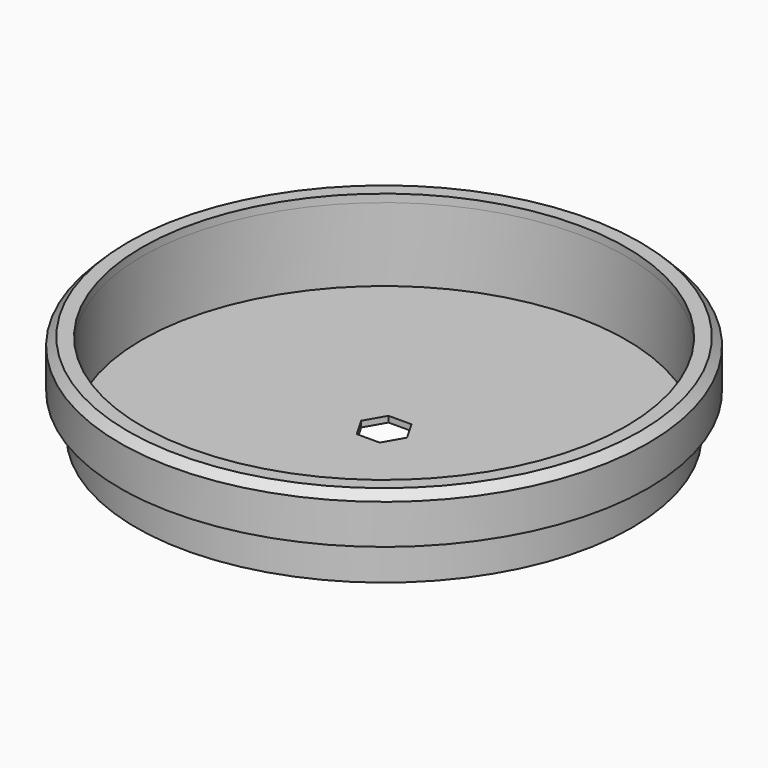
from build123d import *

# Parameters (mm, degrees)
F0_R     = 62.5
F1_DEPTH = 20
F2_T     = -1.5
F3_DEPTH = 25
F4_R     = 66.5
F4_R_2   = 64.5
F4_R_3   = 62.5
F4_R_4   = 61
F5_DEPTH = 2
F6_DEPTH = 10
F7_SIZE  = 1.99999


# Not quite as in the source:
# - a fillet or chamfer is up to 0.001 mm smaller than in the source, because OpenCascade refuses the exact size


with BuildPart() as f1:
    # F0 (on Top) → F1 (new body)
    with BuildSketch(Plane.XY):
        Circle(F0_R)
        Polygon((5.7735026919, 0), (2.8867513459, -5), (-2.8867513459, -5), (-5.7735026919, 0), (-2.8867513459, 5), (2.8867513459, 5), align=None, mode=Mode.SUBTRACT)
        Polygon((-2.8867513459, -5), (2.8867513459, -5), (5.7735026919, 0), (2.8867513459, 5), (-2.8867513459, 5), (-5.7735026919, 0), align=None)
    extrude(amount=F1_DEPTH)

    # F2
    f2_openings = [f1.faces().sort_by_distance(p)[0] for p in [
        (0, 0, 20),
    ]]
    offset(amount=F2_T, openings=f2_openings)

    # F0 (on Top) → F3 (cut)
    with BuildSketch(Plane.XY):
        Polygon((-2.8867513459, -5), (2.8867513459, -5), (5.7735026919, 0), (2.8867513459, 5), (-2.8867513459, 5), (-5.7735026919, 0), align=None)
    extrude(amount=F3_DEPTH, mode=Mode.SUBTRACT)


with BuildPart() as f5:
    # F4 (on face) → F5 (new body)
    with BuildSketch(Plane.XY.offset(20)):
        Circle(F4_R)
        Circle(F4_R_2, mode=Mode.SUBTRACT)
        Circle(F4_R_2)
        Circle(F4_R_3, mode=Mode.SUBTRACT)
        Circle(F4_R_3)
        Circle(F4_R_4, mode=Mode.SUBTRACT)
    extrude(amount=F5_DEPTH)

    # F4 (on face) → F6 (join)
    with BuildSketch(Plane.XY.offset(20)):
        Circle(F4_R)
        Circle(F4_R_2, mode=Mode.SUBTRACT)
    extrude(amount=-F6_DEPTH)

    # F7 (size 2 in the source; OpenCascade refuses exactly that, so slightly less here)
    f7_edges = [f5.edges().sort_by_distance(p)[0] for p in [
        (-66.5, 0, 22),
    ]]
    chamfer(f7_edges, length=F7_SIZE)


solid = Compound([f1.part, f5.part])
